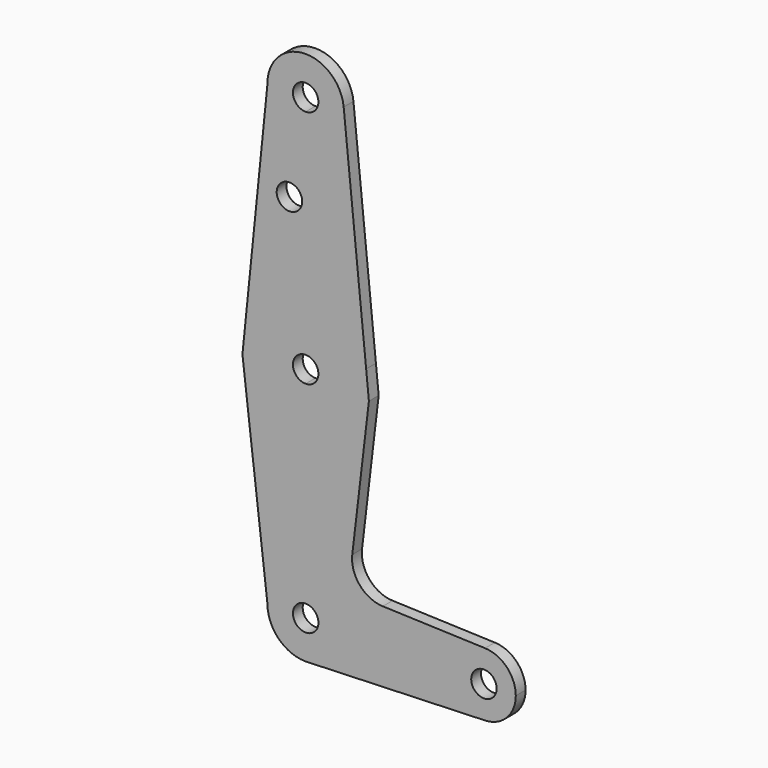
from build123d import *

# Parameters (mm, degrees)
F0_R     = 3.175
F1_DEPTH = 3.048


# Not quite as in the source:
# - a feature of the source that left no trace in its solid (it failed there, or was rolled back) is left out


with BuildPart() as f1:
    # F0 (on Front) → F1 (new body)
    with BuildSketch(Plane.XZ):
        with BuildLine():
            ThreePointArc((9.4771715737, 115.2533330809), (9.5130353789, 114.7772660478), (9.525, 114.3))
            ThreePointArc((9.525, 114.3), (6.7351920908, 107.5648079092), (0, 104.775))
            Line((0, 104.775), (0, 70.485))
            ThreePointArc((0, 70.485), (9.3046760913, 67.4722948122), (15.0777306479, 59.5776617747))
            Line((15.0777306479, 59.5776617747), (9.4771715737, 115.2533330809))
        make_face()
        with BuildLine():
            Line((0, 70.485), (0, 104.775))
            ThreePointArc((0, 104.775), (-6.6805940498, 107.510648916), (-9.5237582055, 114.1461993404))
            Line((-9.5237582055, 114.1461993404), (-15.0673213835, 59.6091450596))
            ThreePointArc((-15.0673213835, 59.6091450596), (-9.2912377318, 67.4820055318), (0, 70.485))
        make_face()
        with Locations((-4.0466510691, 91.1352)):
            Circle(F0_R, mode=Mode.SUBTRACT)
        with BuildLine():
            ThreePointArc((0, 104.775), (6.7351920908, 107.5648079092), (9.525, 114.3))
            ThreePointArc((9.525, 114.3), (9.5130353789, 114.7772660478), (9.4771715737, 115.2533330809))
            ThreePointArc((9.4771715737, 115.2533330809), (-0.5540567285, 123.80887197), (-9.5237582055, 114.1461993404))
            ThreePointArc((-9.5237582055, 114.1461993404), (-6.6805940498, 107.510648916), (0, 104.775))
        make_face()
        with BuildLine():
            ThreePointArc((3.175, 114.3), (2.2450640303, 112.0549359697), (0, 111.125))
            ThreePointArc((0, 111.125), (-2.2450640303, 116.5450640303), (3.175, 114.3))
        make_face(mode=Mode.SUBTRACT)
        with BuildLine():
            Line((15.7650563892, 52.7448935562), (15.0777306479, 59.5776617747))
            ThreePointArc((15.0777306479, 59.5776617747), (9.3046760913, 67.4722948122), (0, 70.485))
            Line((0, 70.485), (0, 57.785))
            ThreePointArc((0, 57.785), (2.2450640303, 56.8550640303), (3.175, 54.61))
            ThreePointArc((3.175, 54.61), (2.2450640303, 52.3649359697), (0, 51.435))
            Line((0, 51.435), (0, 38.735))
            ThreePointArc((0, 38.735), (10.5453084404, 42.743572783), (15.7650563892, 52.7448935562))
        make_face()
        with BuildLine():
            Line((0, 57.785), (0, 70.485))
            ThreePointArc((0, 70.485), (-9.2912377318, 67.4820055318), (-15.0673213835, 59.6091450596))
            Line((-15.0673213835, 59.6091450596), (-15.7650563892, 52.7448935562))
            ThreePointArc((-15.7650563892, 52.7448935562), (-10.5453084404, 42.743572783), (0, 38.735))
            Line((0, 38.735), (0, 51.435))
            ThreePointArc((0, 51.435), (-3.175, 54.61), (0, 57.785))
        make_face()
        with BuildLine():
            ThreePointArc((0, 38.735), (-10.5453084404, 42.743572783), (-15.7650563892, 52.7448935562))
            Line((-15.7650563892, 52.7448935562), (-9.525, 0))
            ThreePointArc((-9.525, 0), (-6.7351920908, 6.7351920908), (0, 9.525))
            Line((0, 9.525), (0, 38.735))
        make_face()
        with BuildLine():
            Line((11.621326375, 17.7194731288), (15.7650563892, 52.7448935562))
            ThreePointArc((15.7650563892, 52.7448935562), (10.5453084404, 42.743572783), (0, 38.735))
            Line((0, 38.735), (0, 9.525))
            ThreePointArc((0, 9.525), (6.7351920908, 6.7351920908), (9.525, 0))
            Line((9.525, 0), (36.5125, 0))
            ThreePointArc((36.5125, 0), (38.9380895153, 5.7116327839), (44.7324052746, 7.9324746146))
            Line((44.7324052746, 7.9324746146), (19.2336094917, 8.8402612478))
            ThreePointArc((19.2336094917, 8.8402612478), (13.480738728, 11.6109066925), (11.621326375, 17.7194731288))
        make_face()
        with BuildLine():
            Line((36.5125, 0), (9.525, 0))
            ThreePointArc((9.525, 0), (6.9705567315, -6.4912990883), (0.6773435479, -9.500885786))
            Line((0.6773435479, -9.500885786), (44.7324052746, -7.9324746146))
            ThreePointArc((44.7324052746, -7.9324746146), (38.9380895153, -5.7116327839), (36.5125, 0))
        make_face()
        with BuildLine():
            ThreePointArc((0, 9.525), (-6.7351920908, 6.7351920908), (-9.525, 0))
            ThreePointArc((-9.525, 0), (-6.7351920908, -6.7351920908), (0, -9.525))
            Line((0, -9.525), (0.6773435479, -9.500885786))
            ThreePointArc((0.6773435479, -9.500885786), (6.9705567315, -6.4912990883), (9.525, 0))
            Line((9.525, 0), (3.175, 0))
            ThreePointArc((3.175, 0), (-2.2450640303, -2.2450640303), (0, 3.175))
            Line((0, 3.175), (0, 9.525))
        make_face()
        with BuildLine():
            ThreePointArc((9.525, 0), (6.7351920908, 6.7351920908), (0, 9.525))
            Line((0, 9.525), (0, 3.175))
            ThreePointArc((0, 3.175), (2.2450640303, 2.2450640303), (3.175, 0))
            Line((3.175, 0), (9.525, 0))
        make_face()
        with BuildLine():
            ThreePointArc((52.3875, 0), (50.1616327839, 5.5119104847), (44.7324052746, 7.9324746146))
            ThreePointArc((44.7324052746, 7.9324746146), (38.9380895153, 5.7116327839), (36.5125, 0))
            ThreePointArc((36.5125, 0), (38.9380895153, -5.7116327839), (44.7324052746, -7.9324746146))
            ThreePointArc((44.7324052746, -7.9324746146), (50.1616327839, -5.5119104847), (52.3875, 0))
        make_face()
        with BuildLine():
            ThreePointArc((47.625, 0), (44.45, -3.175), (41.275, 0))
            ThreePointArc((41.275, 0), (44.45, 3.175), (47.625, 0))
        make_face(mode=Mode.SUBTRACT)
    extrude(amount=F1_DEPTH)


solid = f1.part
